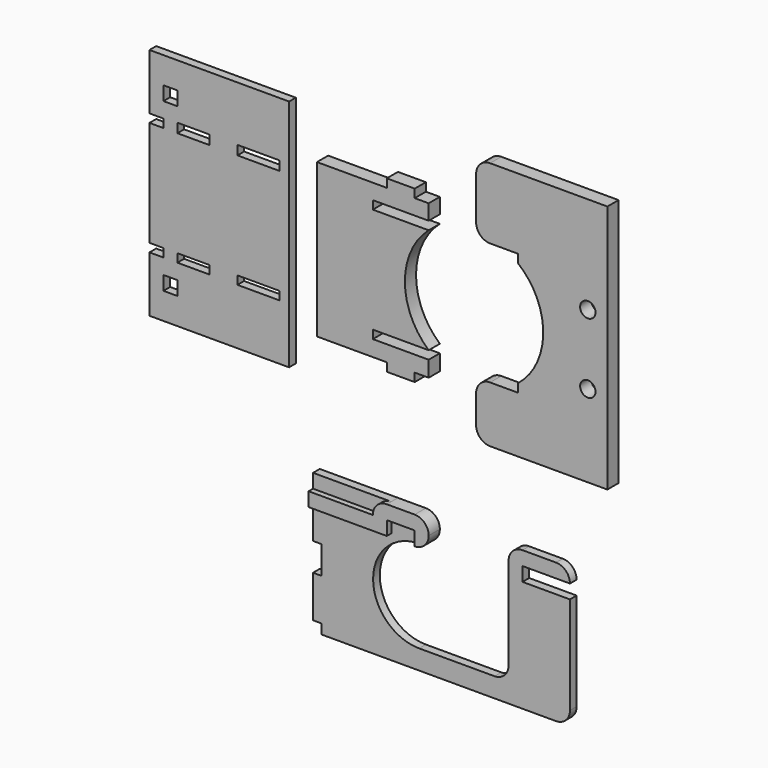
from build123d import *

# Parameters (mm, degrees)
F0_W     = 10
F0_H     = 5
F0_W_2   = 5
F1_DEPTH = 3
F0_W_3   = 11.5
F0_H_2   = 3
F0_H_3   = 3.3244964182
F2_DEPTH = 3
F0_R     = 2.75
F0_W_4   = 17
F0_H_4   = 5.5
F0_H_5   = 5.6787184179
F3_DEPTH = 5
F4_DEPTH = 5
F5_DEPTH = 5
F0_W_5   = 20
F6_DEPTH = 5
F7_DEPTH = 5
F8_R     = 5


with BuildPart() as f1:
    # F0 (on Front) → F1 (new body)
    with BuildSketch(Plane.XZ):
        with BuildLine():
            Line((-76.9379170388, -8.3389794454), (-86.9379170388, -8.3389794454))
            ThreePointArc((-86.9379170388, -8.3389794454), (-90.4734509447, -9.8034455395), (-91.9379170388, -13.3389794454))
            Line((-91.9379170388, -13.3389794454), (-86.9379170388, -13.3389794454))
            Line((-86.9379170388, -13.3389794454), (-76.9379170388, -13.3389794454))
            Line((-76.9379170388, -13.3389794454), (-71.9379170388, -13.3389794454))
            ThreePointArc((-71.9379170388, -13.3389794454), (-73.4023831329, -9.8034455395), (-76.9379170388, -8.3389794454))
        make_face()
        with BuildLine():
            ThreePointArc((-91.9379170388, -13.3389794454), (-90.4734509447, -9.8034455395), (-86.9379170388, -8.3389794454))
            Line((-86.9379170388, -8.3389794454), (-114.9379170388, -8.3389794454))
            Line((-114.9379170388, -8.3389794454), (-114.9379170388, -13.3389794454))
            Line((-114.9379170388, -13.3389794454), (-91.9379170388, -13.3389794454))
        make_face()
        with Locations((-81.9379170388, -15.8389794454)):
            Rectangle(F0_W, F0_H)
        with BuildLine():
            Line((-86.9379170388, -18.3389794454), (-91.9379170388, -18.3389794454))
            Line((-91.9379170388, -18.3389794454), (-111.9379170388, -18.3389794454))
            Line((-111.9379170388, -18.3389794454), (-114.9379170388, -18.3389794454))
            Line((-114.9379170388, -18.3389794454), (-114.9379170388, -29.8389794454))
            Line((-114.9379170388, -29.8389794454), (-111.9379170388, -29.8389794454))
            Line((-111.9379170388, -29.8389794454), (-111.9379170388, -34.8389794454))
            Line((-111.9379170388, -34.8389794454), (-111.9379170388, -39.8389794454))
            Line((-111.9379170388, -39.8389794454), (-114.9379170388, -39.8389794454))
            Line((-114.9379170388, -39.8389794454), (-114.9379170388, -54.8389794454))
            Line((-114.9379170388, -54.8389794454), (-111.9379170388, -54.8389794454))
            Line((-111.9379170388, -54.8389794454), (-111.9379170388, -58.3389794454))
            Line((-111.9379170388, -58.3389794454), (-27.9379170388, -58.3389794454))
            ThreePointArc((-27.9379170388, -58.3389794454), (-24.4023831329, -56.8745133513), (-22.9379170388, -53.3389794454))
            Line((-22.9379170388, -53.3389794454), (-22.9379170388, -18.3389794454))
            Line((-22.9379170388, -18.3389794454), (-39.9379170388, -18.3389794454))
            Line((-39.9379170388, -18.3389794454), (-39.9379170388, -13.3389794454))
            Line((-39.9379170388, -13.3389794454), (-22.9379170388, -13.3389794454))
            ThreePointArc((-22.9379170388, -13.3389794454), (-24.4023831329, -9.8034455395), (-27.9379170388, -8.3389794454))
            Line((-27.9379170388, -8.3389794454), (-39.9379170388, -8.3389794454))
            ThreePointArc((-39.9379170388, -8.3389794454), (-43.4734509447, -9.8034455395), (-44.9379170388, -13.3389794454))
            Line((-44.9379170388, -13.3389794454), (-44.9379170388, -46.3389794454))
            ThreePointArc((-44.9379170388, -46.3389794454), (-46.4023831329, -49.8745133513), (-49.9379170388, -51.3389794454))
            Line((-49.9379170388, -51.3389794454), (-66.9379170388, -51.3389794454))
            Line((-66.9379170388, -51.3389794454), (-76.9379170388, -51.3389794454))
            ThreePointArc((-76.9379170388, -51.3389794454), (-93.4379170388, -34.8389794454), (-76.9379170388, -18.3389794454))
            Line((-76.9379170388, -18.3389794454), (-86.9379170388, -18.3389794454))
        make_face()
        with BuildLine():
            ThreePointArc((-76.9379170388, -18.3389794454), (-73.4023831329, -16.8745133513), (-71.9379170388, -13.3389794454))
            Line((-71.9379170388, -13.3389794454), (-76.9379170388, -13.3389794454))
            Line((-76.9379170388, -13.3389794454), (-76.9379170388, -18.3389794454))
        make_face()
        with Locations((-89.4379170388, -15.8389794454)):
            Rectangle(F0_W_2, F0_H)
    extrude(amount=F1_DEPTH)


with BuildPart() as f2:
    # F0 (on Front) → F2 (new body)
    with BuildSketch(Plane.XZ):
        Polygon((-123.5326989889, 42.1094321907), (-123.5326989889, 105.9307137728), (-172.0326989889, 105.9307137728), (-173.5326989889, 105.9307137728), (-173.5326989889, 85.9307137728), (-172.0326989889, 85.9307137728), (-168.5326989889, 85.9307137728), (-168.5326989889, 82.9307137728), (-172.0326989889, 82.9307137728), (-173.5326989889, 82.9307137728), (-173.5326989889, 45.1094321907), (-172.0326989889, 45.1094321907), (-168.5326989889, 45.1094321907), (-168.5326989889, 42.1094321907), (-172.0326989889, 42.1094321907), (-173.5326989889, 42.1094321907), (-173.5326989889, 22.1094321907), (-172.0326989889, 22.1094321907), (-125.9478926659, 22.1094321907), (-123.5326989889, 22.1094321907), align=None)
        with Locations((-166.0326989889, 34.1094321907)):
            Rectangle(F0_W_2, F0_H, mode=Mode.SUBTRACT)
        with Locations((-157.7826989889, 43.6094321907)):
            Rectangle(F0_W_3, F0_H_2, mode=Mode.SUBTRACT)
        Polygon((-127.0326989889, 42.1094321907), (-142.0326989889, 42.1094321907), (-142.0326989889, 45.1094321907), (-130.5326989889, 45.1094321907), (-127.0326989889, 45.1094321907), align=None, mode=Mode.SUBTRACT)
        with Locations((-157.7826989889, 84.5929619819)):
            Rectangle(F0_W_3, F0_H_3, mode=Mode.SUBTRACT)
        Polygon((-142.0326989889, 86.255210191), (-127.0326989889, 86.255210191), (-127.0326989889, 82.9307137728), (-130.5326989889, 82.9307137728), (-142.0326989889, 82.9307137728), align=None, mode=Mode.SUBTRACT)
        with Locations((-166.0326989889, 93.9307137728)):
            Rectangle(F0_W_2, F0_H, mode=Mode.SUBTRACT)
    extrude(amount=F2_DEPTH)


with BuildPart() as f3:
    # F0 (on Front) → F3 (new body)
    with BuildSketch(Plane.XZ):
        with BuildLine():
            Line((-7.9379170388, 31.4307137728), (-7.9379170388, 96.4307137728))
            Line((-7.9379170388, 96.4307137728), (-7.9379170388, 111.2309247255))
            Line((-7.9379170388, 111.2309247255), (-22.9379170388, 111.2309247255))
            Line((-22.9379170388, 111.2309247255), (-54.9379170388, 111.2309247255))
            Line((-54.9379170388, 111.2309247255), (-54.9379170388, 91.4307137728))
            Line((-54.9379170388, 91.4307137728), (-39.9379170388, 91.4307137728))
            Line((-39.9379170388, 91.4307137728), (-22.9379170388, 91.4307137728))
            Line((-22.9379170388, 91.4307137728), (-22.9379170388, 85.9307137728))
            Line((-22.9379170388, 85.9307137728), (-22.9379170388, 82.9307137728))
            Line((-22.9379170388, 82.9307137728), (-39.9379170388, 82.9307137728))
            ThreePointArc((-39.9379170388, 82.9307137728), (-30.9096430701, 64.0200729817), (-39.9379170388, 45.1094321907))
            Line((-39.9379170388, 45.1094321907), (-22.9379170388, 45.1094321907))
            Line((-22.9379170388, 45.1094321907), (-22.9379170388, 42.1094321907))
            Line((-22.9379170388, 42.1094321907), (-22.9379170388, 36.4307137728))
            Line((-22.9379170388, 36.4307137728), (-39.9379170388, 36.4307137728))
            Line((-39.9379170388, 36.4307137728), (-54.9379170388, 36.4307137728))
            Line((-54.9379170388, 36.4307137728), (-54.9379170388, 21.9877138734))
            Line((-54.9379170388, 21.9877138734), (-22.9379170388, 21.9877138734))
            Line((-22.9379170388, 21.9877138734), (-7.9379170388, 21.9877138734))
            Line((-7.9379170388, 21.9877138734), (-7.9379170388, 31.4307137728))
        make_face()
        with Locations((-14.9379170388, 51.4307137728)):
            Circle(F0_R, mode=Mode.SUBTRACT)
        with Locations((-14.9379170388, 76.4307137728)):
            Circle(F0_R, mode=Mode.SUBTRACT)
        with Locations((-31.4379170388, 84.4307137728)):
            Rectangle(F0_W_4, F0_H_2)
        with Locations((-31.4379170388, 88.6807137728)):
            Rectangle(F0_W_4, F0_H_4)
        Polygon((-39.9379170388, 91.4307137728), (-54.9379170388, 91.4307137728), (-54.9379170388, 85.9307137728), (-44.9379170388, 85.9307137728), (-39.9379170388, 85.9307137728), align=None)
        with Locations((-31.4379170388, 43.6094321907)):
            Rectangle(F0_W_4, F0_H_2)
        with Locations((-31.4379170388, 39.2700729817)):
            Rectangle(F0_W_4, F0_H_5)
        Polygon((-54.9379170388, 42.1094321907), (-54.9379170388, 36.4307137728), (-39.9379170388, 36.4307137728), (-39.9379170388, 42.1094321907), (-44.9379170388, 42.1094321907), align=None)
    extrude(amount=F3_DEPTH)

    # F8
    f8_edges = [f3.edges().sort_by_distance(p)[0] for p in [
        (-54.937917, -2.5, 42.109432),
        (-54.937917, -2.5, 85.930714),
        (-54.937917, -2.5, 21.987714),
        (-54.937917, -2.5, 111.230925),
    ]]
    fillet(f8_edges, radius=F8_R)


with BuildPart() as f4:
    # F0 (on Front) → F4 (new body)
    with BuildSketch(Plane.XZ):
        Polygon((-86.9379170388, 85.9307137728), (-71.9379170388, 85.9307137728), (-71.9379170388, 91.4307137728), (-76.9379170388, 91.4307137728), (-86.9379170388, 91.4307137728), (-91.9379170388, 91.4307137728), (-111.9379170388, 91.4307137728), (-111.9379170388, 85.9307137728), (-91.9379170388, 85.9307137728), align=None)
        Polygon((-71.9379170388, 36.4307137728), (-71.9379170388, 42.1094321907), (-86.9379170388, 42.1094321907), (-91.9379170388, 42.1094321907), (-111.9379170388, 42.1094321907), (-111.9379170388, 36.4307137728), (-86.9379170388, 36.4307137728), (-76.9379170388, 36.4307137728), align=None)
        with Locations((-89.4379170388, 84.4307137728)):
            Rectangle(F0_W_2, F0_H_2)
        with BuildLine():
            ThreePointArc((-71.9379170388, 45.1094321907), (-80.4638719585, 64.0200729817), (-71.9379170388, 82.9307137728))
            Line((-71.9379170388, 82.9307137728), (-86.9379170388, 82.9307137728))
            Line((-86.9379170388, 82.9307137728), (-91.9379170388, 82.9307137728))
            Line((-91.9379170388, 82.9307137728), (-111.9379170388, 82.9307137728))
            Line((-111.9379170388, 82.9307137728), (-111.9379170388, 80.9307137728))
            Line((-111.9379170388, 80.9307137728), (-111.9379170388, 45.1094321907))
            Line((-111.9379170388, 45.1094321907), (-91.9379170388, 45.1094321907))
            Line((-91.9379170388, 45.1094321907), (-86.9379170388, 45.1094321907))
            Line((-86.9379170388, 45.1094321907), (-71.9379170388, 45.1094321907))
        make_face()
        with Locations((-89.4379170388, 43.6094321907)):
            Rectangle(F0_W_2, F0_H_2)
    extrude(amount=F4_DEPTH)

    # F0 (on Front) → F6 (join)
    with BuildSketch(Plane.XZ):
        Polygon((-76.9379170388, 33.4307137728), (-76.9379170388, 36.4307137728), (-86.9379170388, 36.4307137728), (-86.9379170388, 33.4307137728), (-78.4176960588, 33.4307137728), align=None)
        with Locations((-81.9379170388, 92.9307137728)):
            Rectangle(F0_W, F0_H_2)
        with Locations((-101.9379170388, 84.4307137728)):
            Rectangle(F0_W_5, F0_H_2)
        with Locations((-101.9379170388, 43.6094321907)):
            Rectangle(F0_W_5, F0_H_2)
        with Locations((-89.4379170388, 84.4307137728)):
            Rectangle(F0_W_2, F0_H_2)
        with Locations((-89.4379170388, 43.6094321907)):
            Rectangle(F0_W_2, F0_H_2)
    extrude(amount=F6_DEPTH)

    # F0 (on Front) → F7 (cut)
    with BuildSketch(Plane.XZ):
        with Locations((-89.4379170388, 84.4307137728)):
            Rectangle(F0_W_2, F0_H_2)
        with Locations((-89.4379170388, 43.6094321907)):
            Rectangle(F0_W_2, F0_H_2)
    extrude(amount=F7_DEPTH, mode=Mode.SUBTRACT)


with BuildPart() as f4b:
    # F0 (on Front) → F4, piece 2 (new body)
    with BuildSketch(Plane.XZ):
        with BuildLine():
            Line((-76.9379170388, -8.3389794454), (-86.9379170388, -8.3389794454))
            ThreePointArc((-86.9379170388, -8.3389794454), (-90.4734509447, -9.8034455395), (-91.9379170388, -13.3389794454))
            Line((-91.9379170388, -13.3389794454), (-86.9379170388, -13.3389794454))
            Line((-86.9379170388, -13.3389794454), (-76.9379170388, -13.3389794454))
            Line((-76.9379170388, -13.3389794454), (-71.9379170388, -13.3389794454))
            ThreePointArc((-71.9379170388, -13.3389794454), (-73.4023831329, -9.8034455395), (-76.9379170388, -8.3389794454))
        make_face()
    extrude(amount=F4_DEPTH)

    # F0 (on Front) → F4, piece 3 (join)
    with BuildSketch(Plane.XZ):
        Polygon((-91.9379170388, -18.3389794454), (-91.9379170388, -13.3389794454), (-114.9379170388, -13.3389794454), (-114.9379170388, -18.3389794454), (-111.9379170388, -18.3389794454), align=None)
    extrude(amount=F4_DEPTH)

    # F0 (on Front) → F5 (join)
    with BuildSketch(Plane.XZ):
        Polygon((-91.9379170388, -18.3389794454), (-91.9379170388, -13.3389794454), (-114.9379170388, -13.3389794454), (-114.9379170388, -18.3389794454), (-111.9379170388, -18.3389794454), align=None)
        with Locations((-89.4379170388, -15.8389794454)):
            Rectangle(F0_W_2, F0_H)
        with BuildLine():
            Line((-76.9379170388, -8.3389794454), (-86.9379170388, -8.3389794454))
            ThreePointArc((-86.9379170388, -8.3389794454), (-90.4734509447, -9.8034455395), (-91.9379170388, -13.3389794454))
            Line((-91.9379170388, -13.3389794454), (-86.9379170388, -13.3389794454))
            Line((-86.9379170388, -13.3389794454), (-76.9379170388, -13.3389794454))
            Line((-76.9379170388, -13.3389794454), (-71.9379170388, -13.3389794454))
            ThreePointArc((-71.9379170388, -13.3389794454), (-73.4023831329, -9.8034455395), (-76.9379170388, -8.3389794454))
        make_face()
        with BuildLine():
            ThreePointArc((-76.9379170388, -18.3389794454), (-73.4023831329, -16.8745133513), (-71.9379170388, -13.3389794454))
            Line((-71.9379170388, -13.3389794454), (-76.9379170388, -13.3389794454))
            Line((-76.9379170388, -13.3389794454), (-76.9379170388, -18.3389794454))
        make_face()
    extrude(amount=F5_DEPTH)


solid = Compound([f1.part, f2.part, f3.part, f4.part, f4b.part])
